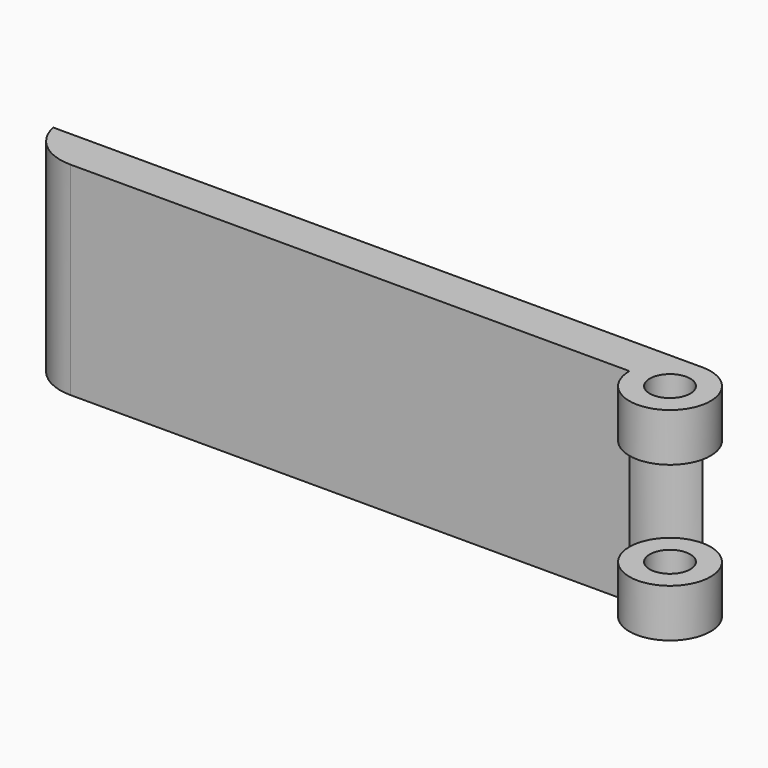
from build123d import *

# Parameters (mm, degrees)
F0_R        = 2
F1_DEPTH    = 10
F2_DEPTH    = 5.25
F3_T1_DEPTH = 44.4948974279


# Not quite as in the source:
# - a fillet or chamfer that OpenCascade refuses, or shapes differently, is made with other operations: its cross-section is extruded or revolved along the edge and cut away or added


with BuildPart() as f1:
    # F0 (on Top) → F1 (new body, symmetric)
    with BuildSketch(Plane.XY):
        with BuildLine():
            Line((64, 0), (0, 0))
            Line((0, 0), (0, -4))
            Line((0, -4), (60, -4))
            ThreePointArc((60, -4), (61.1715728753, -1.1715728753), (64, 0))
        make_face()
        with BuildLine():
            ThreePointArc((68, -4), (66.8284271247, -1.1715728753), (64, 0))
            ThreePointArc((64, 0), (61.1715728753, -1.1715728753), (60, -4))
            ThreePointArc((60, -4), (64, -8), (68, -4))
        make_face()
        with Locations((64, -4)):
            Circle(F0_R, mode=Mode.SUBTRACT)
    extrude(amount=F1_DEPTH, both=True)

    # F0 (on Top) → F2 (cut, symmetric)
    with BuildSketch(Plane.XY):
        with BuildLine():
            ThreePointArc((68, -4), (66.8284271247, -1.1715728753), (64, 0))
            ThreePointArc((64, 0), (61.1715728753, -1.1715728753), (60, -4))
            ThreePointArc((60, -4), (64, -8), (68, -4))
        make_face()
        with Locations((64, -4)):
            Circle(F0_R, mode=Mode.SUBTRACT)
    extrude(amount=F2_DEPTH, both=True, mode=Mode.SUBTRACT)

    # F3: fillet of radius 5 on 1 edges, made by hand

    # F3_s2 → F3_t1 (cut)
    with BuildSketch(Plane.XY.offset(-22.2474487139)):
        with BuildLine():
            ThreePointArc((4.8989794856, -4), (1.7367018254, -2.8729833462), (0, 0))
            Line((0, 0), (0, -4))
            Line((0, -4), (4.8989794856, -4))
        make_face()
    extrude(amount=F3_T1_DEPTH, mode=Mode.SUBTRACT)


solid = f1.part
